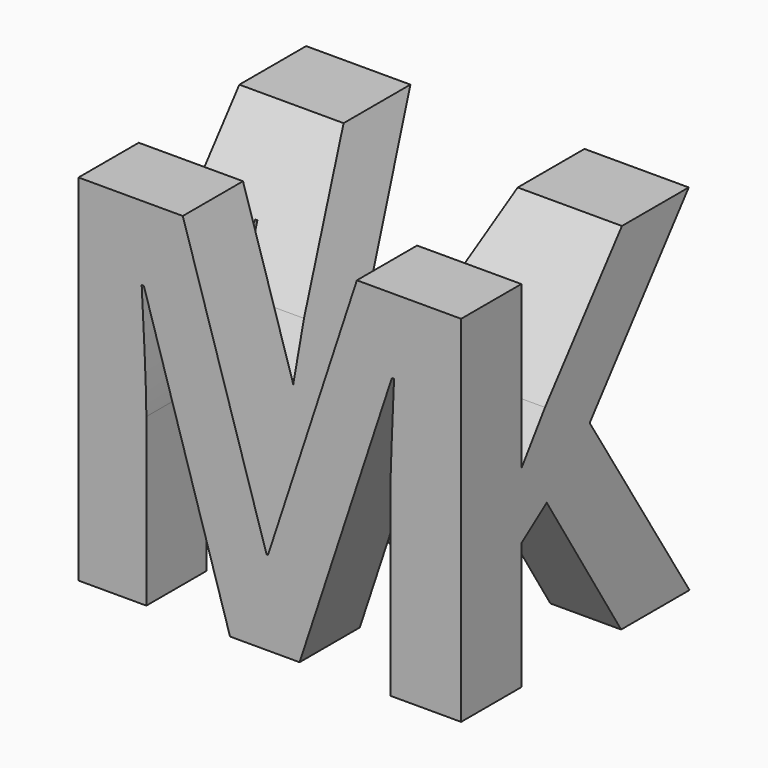
from build123d import *

# Parameters (mm, degrees)
F0_TEXT_SIZE = 55.5555555556
F1_DEPTH     = 40
F2_TEXT_SIZE = 55.0853587963
F3_DEPTH     = 42.3958333333


# Not quite as in the source:
# - a feature of the source that left no trace in its solid (it failed there, or was rolled back) is left out
# - Text() gives the source's letters only with a copy of the font that has no kerning and outlines rounded to 1/6400 em; it was checked with that copy


with BuildPart() as f1:
    # F0 (on Front) → F1 (new body)
    with BuildSketch(Plane.XZ):
        with Locations((0, 0)):
            Text('M', F0_TEXT_SIZE, font='Open Sans', font_style=FontStyle.BOLD, text_align=(TextAlign.LEFT, TextAlign.BOTTOM))
    extrude(amount=-F1_DEPTH)


with BuildPart() as f3:
    # F2 (on face) → F3 (new body, through all)
    with BuildSketch(Plane.YZ.offset(47.3871527778)):
        with Locations((0, 0)):
            Text('K', F2_TEXT_SIZE, font='Open Sans', font_style=FontStyle.BOLD, text_align=(TextAlign.LEFT, TextAlign.BOTTOM))
    extrude(amount=-F3_DEPTH)

    # F4: intersect F1
    add(f1.part, mode=Mode.INTERSECT)


solid = f3.part
